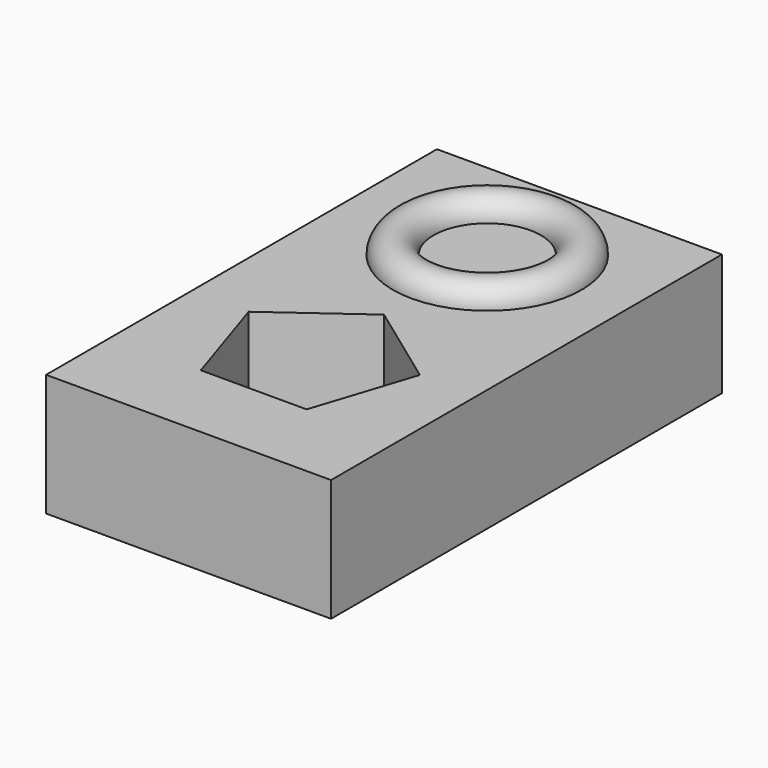
from build123d import *

# Parameters (mm, degrees)
F0_W     = 35
F0_H     = 60
F1_DEPTH = 15
F3_DEPTH = 25


with BuildPart() as f1:
    # F0 (on Top) → F1 (new body)
    with BuildSketch(Plane.XY):
        with Locations((17.5, 30)):
            Rectangle(F0_W, F0_H)
    extrude(amount=F1_DEPTH)

    # F2 (on face) → F3 (cut)
    with BuildSketch(Plane.XY.offset(15)):
        Polygon((23.9983939247, 10), (28.0146222424, 22.360679775), (17.5, 30), (6.9853777576, 22.360679775), (11.0016060753, 10), align=None)
    extrude(amount=-F3_DEPTH, mode=Mode.SUBTRACT)

    # F5 (on mid) → F6 (revolve)
    with BuildSketch(Plane.YZ.offset(17.5)):
        with BuildLine():
            Line((34.2611013353, 15), (39.2611013353, 15))
            ThreePointArc((39.2611013353, 15), (36.7611013353, 17.5), (34.2611013353, 15))
        make_face()
        with BuildLine():
            ThreePointArc((34.2611013353, 15), (36.7611013353, 12.5), (39.2611013353, 15))
            Line((39.2611013353, 15), (34.2611013353, 15))
        make_face()
    revolve(axis=Axis((17.5, 45.8512790501, 18.8291036189), (0, 0, 1)))


solid = f1.part
